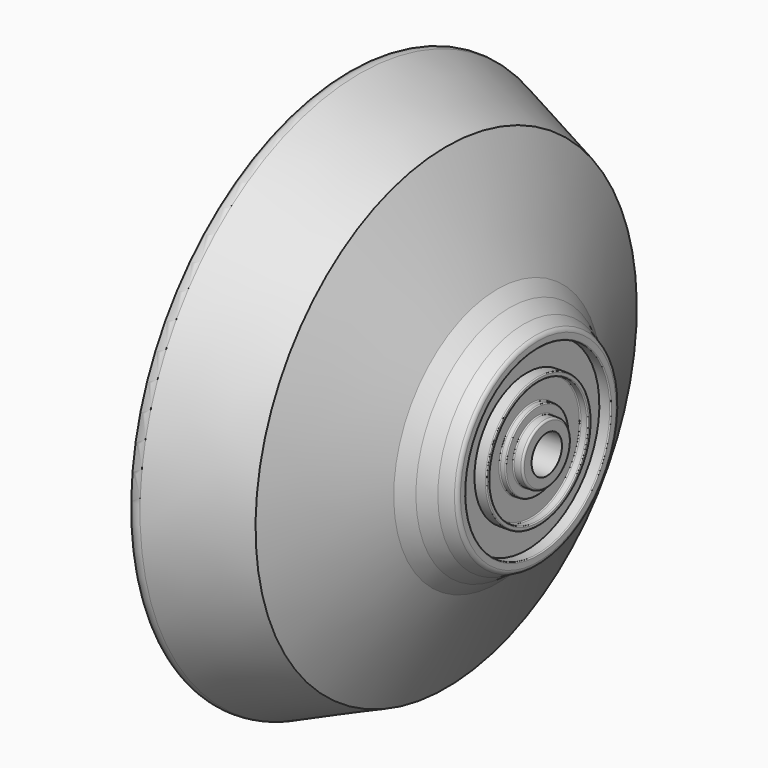
from build123d import *

# Parameters (mm, degrees)
F2_R = 0.1
F3_R = 0.2
F4_R = 1
F5_R = 10
F6_R = 0.5


with BuildPart() as f1:
    # F0 (on Front) → F1 (revolve)
    with BuildSketch(Plane.XZ):
        with BuildLine():
            Line((-4.2, 2), (-1.4, 2))
            Line((-1.4, 2), (-1.4, 3.17))
            Line((-1.4, 3.17), (-2.4, 3.17))
            Line((-2.4, 3.17), (-2.4, 4.15))
            Line((-2.4, 4.15), (-3.05, 4.15))
            Line((-3.05, 4.15), (-3.05, 6.45))
            Line((-3.05, 6.45), (-2.25, 6.45))
            Line((-2.25, 6.45), (-2.25, 6.9))
            Line((-2.25, 6.9), (-3.5, 6.9))
            Line((-3.5, 6.9), (-3.5, 9.55))
            Line((-3.5, 9.55), (-2.3, 9.55))
            Line((-2.3, 9.55), (-2.3, 10.55))
            Line((-2.3, 10.55), (-3.8220669191, 11.3141352547))
            Line((-3.8220669191, 11.3141352547), (-5.3048291735, 12.3523765626))
            Line((-5.3048291735, 12.3523765626), (-6.6017600859, 13.649307475))
            Line((-6.6017600859, 13.649307475), (-12.0003940538, 25.1019764692))
            Line((-12.0003940538, 25.1019764692), (-22.5, 29.5))
            Line((-22.5, 29.5), (-22.5, 23.4155036587))
            ThreePointArc((-22.5, 23.4155036587), (-22.0466673369, 22.578153778), (-21.0976903546, 22.5))
            Line((-21.0976903546, 22.5), (-20.5097097557, 22.7583826553))
            ThreePointArc((-20.5097097557, 22.7583826553), (-14.712886985, 22.9204669678), (-10.446965114, 18.9921930276))
            Line((-10.446965114, 18.9921930276), (-7.5, 12.7404974711))
            Line((-7.5, 12.7404974711), (-7.5, 8))
            Line((-7.5, 8), (-4.7, 8))
            Line((-4.7, 8), (-4.7, 6.1651659198))
            Line((-4.7, 6.1651659198), (-4.25, 6.1651659198))
            Line((-4.25, 6.1651659198), (-4.25, 3.17))
            Line((-4.25, 3.17), (-5.1078278272, 2.4200506077))
            Line((-5.1078278272, 2.4200506077), (-6.3, 0))
            Line((-6.3, 0), (-5.1852456548, 0))
            Line((-5.1852456548, 0), (-4.2, 2))
        make_face()
    revolve(axis=Axis((-5.7426228274, 0, 0), (-1, 0, 0)))

    # F2
    f2_edges = [f1.edges().sort_by_distance(p)[0] for p in [
        (-2.4, 0, -4.15),
        (-3.05, 0, -4.15),
        (-2.25, 0, -6.45),
        (-2.25, 0, -6.9),
        (-2.3, 0, -9.55),
        (-3.05, 0, -6.45),
        (-2.4, 0, -3.17),
    ]]
    fillet(f2_edges, radius=F2_R)

    # F3
    f3_edges = [f1.edges().sort_by_distance(p)[0] for p in [
        (-1.4, 0, -3.17),
    ]]
    fillet(f3_edges, radius=F3_R)

    # F4
    f4_edges = [f1.edges().sort_by_distance(p)[0] for p in [
        (-22.5, 0, -29.5),
    ]]
    fillet(f4_edges, radius=F4_R)

    # F5
    f5_edges = [f1.edges().sort_by_distance(p)[0] for p in [
        (-7.5, 0, -12.740497),
    ]]
    fillet(f5_edges, radius=F5_R)

    # F6
    f6_edges = [f1.edges().sort_by_distance(p)[0] for p in [
        (-2.3, 0, -10.55),
    ]]
    fillet(f6_edges, radius=F6_R)


solid = f1.part
